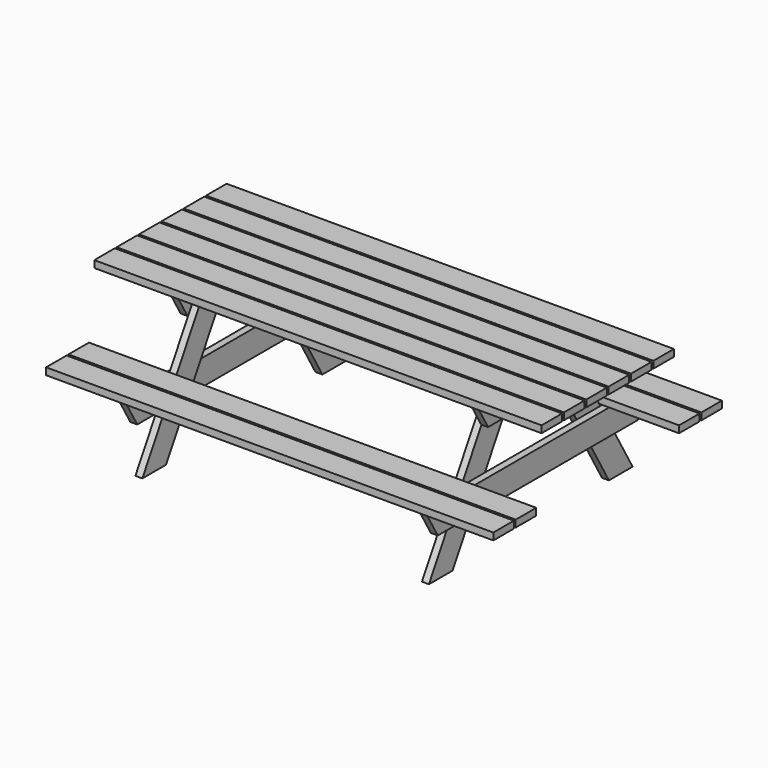
from build123d import *

# Parameters (mm, degrees)
F1_DEPTH      = 38.1
F3_DEPTH      = 38.1
F4_W          = 139.7
F4_H          = 38.1
F5_DEPTH      = 381
F5_DEPTH_BACK = 2057.4


# Not quite as in the source:
# - a pattern or mirror of a feature is missing from the dataset's text; its kind, count and spacing are read off the source's solid


with BuildPart() as f1:
    # F0 (on Right) → F1 (new body)
    with BuildSketch(Plane.YZ):
        Polygon((-254, 762), (-693.9409051225, 0), (-532.6292399109, 0), (-92.6883347884, 762), align=None)
    extrude(amount=F1_DEPTH)


with BuildPart() as f1b:
    # F0 (on Right) → F1, piece 2 (new body)
    with BuildSketch(Plane.YZ):
        Polygon((254, 762), (92.6883347884, 762), (532.6292399109, 0), (693.9409051225, 0), align=None)
    extrude(amount=F1_DEPTH)


with BuildPart() as f1_copies_1:
    # F1_copies: instance of F1
    add(f1.part.mirror(Plane(origin=(-762, 0, 0), x_dir=(0, 0, -1), z_dir=(-1, 0, 0))))


with BuildPart() as f1_2_copies_1:
    # F1_2_copies: instance of F1b
    add(f1b.part.mirror(Plane(origin=(-762, 0, 0), x_dir=(0, 0, -1), z_dir=(-1, 0, 0))))


with BuildPart() as f1_1:
    add(f1.part)

    add(f1b.part)  # F3 merges F1b
    # F2 (on face) → F3 (join)
    with BuildSketch(Plane.YZ.offset(38.1)):
        Polygon((762, 381), (-762, 381), (-681.3441673942, 241.3), (681.3441673942, 241.3), align=None)
        Polygon((419.1, 762), (-419.1, 762), (-338.4441673942, 622.3), (338.4441673942, 622.3), align=None)
    f3 = extrude(amount=F3_DEPTH)

    # F3_copies: F3 across plane
    add(f3.mirror(Plane(origin=(-762, 0, 0), x_dir=(0, 0, -1), z_dir=(-1, 0, 0))))

    add(f1_copies_1.part)  # F5 merges F1_copies_1

    add(f1_2_copies_1.part)  # F5 merges F1_2_copies_1
    # F4 (on face) → F5 (join, two sides)
    with BuildSketch(Plane.YZ.offset(76.2)) as f5_sk:
        with Locations((-708.9204525612, 400.05)):
            Rectangle(F4_W, F4_H)
        with Locations((-556.5204525612, 400.05)):
            Rectangle(F4_W, F4_H)
        with Locations((556.5204525612, 400.05)):
            Rectangle(F4_W, F4_H)
        with Locations((708.9204525612, 400.05)):
            Rectangle(F4_W, F4_H)
        with Locations((-380.4596342087, 781.05)):
            Rectangle(F4_W, F4_H)
        with Locations((-228.0596342087, 781.05)):
            Rectangle(F4_W, F4_H)
        with Locations((-75.6596342087, 781.05)):
            Rectangle(F4_W, F4_H)
        with Locations((76.7403657913, 781.05)):
            Rectangle(F4_W, F4_H)
        with Locations((229.1403657913, 781.05)):
            Rectangle(F4_W, F4_H)
        with Locations((381.5403657913, 781.05)):
            Rectangle(F4_W, F4_H)
    extrude(amount=F5_DEPTH)
    extrude(f5_sk.sketch, amount=-F5_DEPTH_BACK)


solid = f1_1.part
